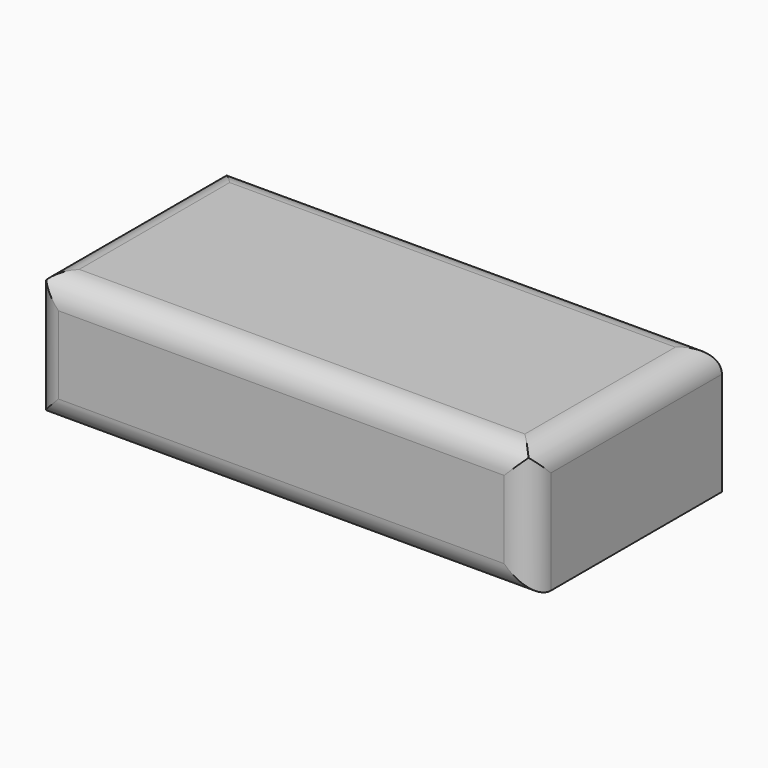
from build123d import *

# Parameters (mm, degrees)
F0_W        = 97.5638087839
F0_H        = 47.0372922719
F1_DEPTH    = 25.4
F2_R        = 5.08
F3_T1_DEPTH = 67.3572922719
F3_T3_DEPTH = 122.9638087839


# Not quite as in the source:
# - a fillet or chamfer that OpenCascade refuses, or shapes differently, is made with other operations: its cross-section is extruded or revolved along the edge and cut away or added


with BuildPart() as f1:
    # F0 (on Top) → F1 (new body)
    with BuildSketch(Plane.XY):
        with Locations((25.0818403438, 62.9095640033)):
            Rectangle(F0_W, F0_H)
    extrude(amount=F1_DEPTH)

    # F2
    f2_edges = [f1.edges().sort_by_distance(p)[0] for p in [
        (73.863745, 39.390918, 12.7),
        (25.08184, 39.390918, 25.4),
        (-23.700064, 39.390918, 12.7),
        (25.08184, 39.390918, 0),
    ]]
    fillet(f2_edges, radius=F2_R)

    # F3: fillet of radius 5.08 on 8 edges, made by hand

    # F3_s2 → F3_t1 (cut)
    with BuildSketch(Plane.XZ.offset(-99.1282101393)):
        with BuildLine():
            ThreePointArc((73.8637447357, 20.32), (72.3758471841, 23.9121024484), (68.7837447357, 25.4))
            Line((68.7837447357, 25.4), (73.8637447357, 25.4))
            Line((73.8637447357, 25.4), (73.8637447357, 20.32))
        make_face()
        with BuildLine():
            ThreePointArc((-18.6200640482, 25.4), (-22.2121664966, 23.9121024484), (-23.7000640482, 20.32))
            Line((-23.7000640482, 20.32), (-23.7000640482, 25.4))
            Line((-23.7000640482, 25.4), (-18.6200640482, 25.4))
        make_face()
    extrude(amount=F3_T1_DEPTH, mode=Mode.SUBTRACT)

    # F3_s4 → F3_t3 (cut)
    with BuildSketch(Plane.YZ.offset(-36.4000640482)):
        with BuildLine():
            ThreePointArc((86.4282101393, 20.32), (84.9403125877, 23.9121024484), (81.3482101393, 25.4))
            Line((81.3482101393, 25.4), (86.4282101393, 25.4))
            Line((86.4282101393, 25.4), (86.4282101393, 20.32))
        make_face()
    extrude(amount=F3_T3_DEPTH, mode=Mode.SUBTRACT)


solid = f1.part
